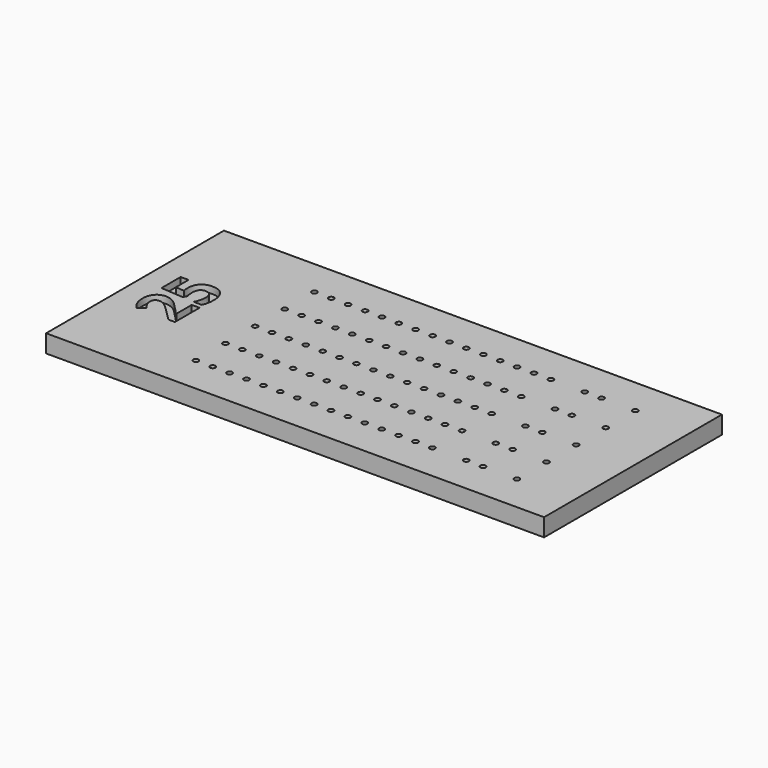
from build123d import *

# Parameters (mm, degrees)
F0_W         = 112
F0_H         = 50
F1_DEPTH     = 4
F2_TEXT_SIZE = 13.8888888889
F3_DEPTH     = 1.5
F4_R         = 0.6
F5_DEPTH     = 4


# Not quite as in the source:
# - Text() gives the source's letters only with a copy of the font that has no kerning and outlines rounded to 1/6400 em; it was checked with that copy


with BuildPart() as f1:
    # F0 (on Top) → F1 (new body)
    with BuildSketch(Plane.XY):
        with Locations((12.8412768841, 3.3350909071)):
            Rectangle(F0_W, F0_H)
    extrude(amount=F1_DEPTH)

    # F2 (on face) → F3 (cut)
    with BuildSketch(Plane.XY.offset(4)):
        with Locations(Location((-28.1587231159, -4.7477215929), (0, 0, 90))):
            Text('25', F2_TEXT_SIZE, font='Open Sans', font_style=FontStyle.BOLD, text_align=(TextAlign.LEFT, TextAlign.BOTTOM))
    extrude(amount=-F3_DEPTH, mode=Mode.SUBTRACT)

    # F4 (on face) → F5 (cut, through all)
    with BuildSketch(Plane.XY.offset(4)):
        with Locations((-16.1587231159, 20.0050909071)):
            Circle(F4_R)
        with Locations((-12.3587231159, 20.0050909071)):
            Circle(F4_R)
        with Locations((-8.5587231159, 20.0050909071)):
            Circle(F4_R)
        with Locations((-4.7587231159, 20.0050909071)):
            Circle(F4_R)
        with Locations((-0.9587231159, 20.0050909071)):
            Circle(F4_R)
        with Locations((2.8412768841, 20.0050909071)):
            Circle(F4_R)
        with Locations((6.6412768841, 20.0050909071)):
            Circle(F4_R)
        with Locations((10.4412768841, 20.0050909071)):
            Circle(F4_R)
        with Locations((14.2412768841, 20.0050909071)):
            Circle(F4_R)
        with Locations((18.0412768841, 20.0050909071)):
            Circle(F4_R)
        with Locations((21.8412768841, 20.0050909071)):
            Circle(F4_R)
        with Locations((25.6412768841, 20.0050909071)):
            Circle(F4_R)
        with Locations((29.4412768841, 20.0050909071)):
            Circle(F4_R)
        with Locations((33.2412768841, 20.0050909071)):
            Circle(F4_R)
        with Locations((37.0412768841, 20.0050909071)):
            Circle(F4_R)
        with Locations((44.6412768841, 20.0050909071)):
            Circle(F4_R)
        with Locations((48.4412768841, 20.0050909071)):
            Circle(F4_R)
        with Locations((56.0412768841, 20.0050909071)):
            Circle(F4_R)
        with Locations((-16.1587231159, 11.6750909071)):
            Circle(F4_R)
        with Locations((-12.3587231159, 11.6750909071)):
            Circle(F4_R)
        with Locations((-8.5587231159, 11.6750909071)):
            Circle(F4_R)
        with Locations((-4.7587231159, 11.6750909071)):
            Circle(F4_R)
        with Locations((-0.9587231159, 11.6750909071)):
            Circle(F4_R)
        with Locations((2.8412768841, 11.6750909071)):
            Circle(F4_R)
        with Locations((6.6412768841, 11.6750909071)):
            Circle(F4_R)
        with Locations((10.4412768841, 11.6750909071)):
            Circle(F4_R)
        with Locations((14.2412768841, 11.6750909071)):
            Circle(F4_R)
        with Locations((18.0412768841, 11.6750909071)):
            Circle(F4_R)
        with Locations((21.8412768841, 11.6750909071)):
            Circle(F4_R)
        with Locations((25.6412768841, 11.6750909071)):
            Circle(F4_R)
        with Locations((29.4412768841, 11.6750909071)):
            Circle(F4_R)
        with Locations((33.2412768841, 11.6750909071)):
            Circle(F4_R)
        with Locations((37.0412768841, 11.6750909071)):
            Circle(F4_R)
        with Locations((44.6412768841, 11.6750909071)):
            Circle(F4_R)
        with Locations((48.4412768841, 11.6750909071)):
            Circle(F4_R)
        with Locations((56.0412768841, 11.6750909071)):
            Circle(F4_R)
        with Locations((-16.1587231159, 3.3450909071)):
            Circle(F4_R)
        with Locations((-12.3587231159, 3.3450909071)):
            Circle(F4_R)
        with Locations((-8.5587231159, 3.3450909071)):
            Circle(F4_R)
        with Locations((-4.7587231159, 3.3450909071)):
            Circle(F4_R)
        with Locations((-0.9587231159, 3.3450909071)):
            Circle(F4_R)
        with Locations((2.8412768841, 3.3450909071)):
            Circle(F4_R)
        with Locations((6.6412768841, 3.3450909071)):
            Circle(F4_R)
        with Locations((10.4412768841, 3.3450909071)):
            Circle(F4_R)
        with Locations((14.2412768841, 3.3450909071)):
            Circle(F4_R)
        with Locations((18.0412768841, 3.3450909071)):
            Circle(F4_R)
        with Locations((21.8412768841, 3.3450909071)):
            Circle(F4_R)
        with Locations((25.6412768841, 3.3450909071)):
            Circle(F4_R)
        with Locations((29.4412768841, 3.3450909071)):
            Circle(F4_R)
        with Locations((33.2412768841, 3.3450909071)):
            Circle(F4_R)
        with Locations((37.0412768841, 3.3450909071)):
            Circle(F4_R)
        with Locations((44.6412768841, 3.3450909071)):
            Circle(F4_R)
        with Locations((48.4412768841, 3.3450909071)):
            Circle(F4_R)
        with Locations((56.0412768841, 3.3450909071)):
            Circle(F4_R)
        with Locations((-16.1587231159, -4.9849090929)):
            Circle(F4_R)
        with Locations((-12.3587231159, -4.9849090929)):
            Circle(F4_R)
        with Locations((-8.5587231159, -4.9849090929)):
            Circle(F4_R)
        with Locations((-4.7587231159, -4.9849090929)):
            Circle(F4_R)
        with Locations((-0.9587231159, -4.9849090929)):
            Circle(F4_R)
        with Locations((2.8412768841, -4.9849090929)):
            Circle(F4_R)
        with Locations((6.6412768841, -4.9849090929)):
            Circle(F4_R)
        with Locations((10.4412768841, -4.9849090929)):
            Circle(F4_R)
        with Locations((14.2412768841, -4.9849090929)):
            Circle(F4_R)
        with Locations((18.0412768841, -4.9849090929)):
            Circle(F4_R)
        with Locations((21.8412768841, -4.9849090929)):
            Circle(F4_R)
        with Locations((25.6412768841, -4.9849090929)):
            Circle(F4_R)
        with Locations((29.4412768841, -4.9849090929)):
            Circle(F4_R)
        with Locations((33.2412768841, -4.9849090929)):
            Circle(F4_R)
        with Locations((37.0412768841, -4.9849090929)):
            Circle(F4_R)
        with Locations((44.6412768841, -4.9849090929)):
            Circle(F4_R)
        with Locations((48.4412768841, -4.9849090929)):
            Circle(F4_R)
        with Locations((56.0412768841, -4.9849090929)):
            Circle(F4_R)
        with Locations((-16.1587231159, -13.3149090929)):
            Circle(F4_R)
        with Locations((-12.3587231159, -13.3149090929)):
            Circle(F4_R)
        with Locations((-8.5587231159, -13.3149090929)):
            Circle(F4_R)
        with Locations((-4.7587231159, -13.3149090929)):
            Circle(F4_R)
        with Locations((-0.9587231159, -13.3149090929)):
            Circle(F4_R)
        with Locations((2.8412768841, -13.3149090929)):
            Circle(F4_R)
        with Locations((6.6412768841, -13.3149090929)):
            Circle(F4_R)
        with Locations((10.4412768841, -13.3149090929)):
            Circle(F4_R)
        with Locations((14.2412768841, -13.3149090929)):
            Circle(F4_R)
        with Locations((18.0412768841, -13.3149090929)):
            Circle(F4_R)
        with Locations((21.8412768841, -13.3149090929)):
            Circle(F4_R)
        with Locations((25.6412768841, -13.3149090929)):
            Circle(F4_R)
        with Locations((29.4412768841, -13.3149090929)):
            Circle(F4_R)
        with Locations((33.2412768841, -13.3149090929)):
            Circle(F4_R)
        with Locations((37.0412768841, -13.3149090929)):
            Circle(F4_R)
        with Locations((44.6412768841, -13.3149090929)):
            Circle(F4_R)
        with Locations((48.4412768841, -13.3149090929)):
            Circle(F4_R)
        with Locations((56.0412768841, -13.3149090929)):
            Circle(F4_R)
    extrude(amount=-F5_DEPTH, mode=Mode.SUBTRACT)


solid = f1.part
